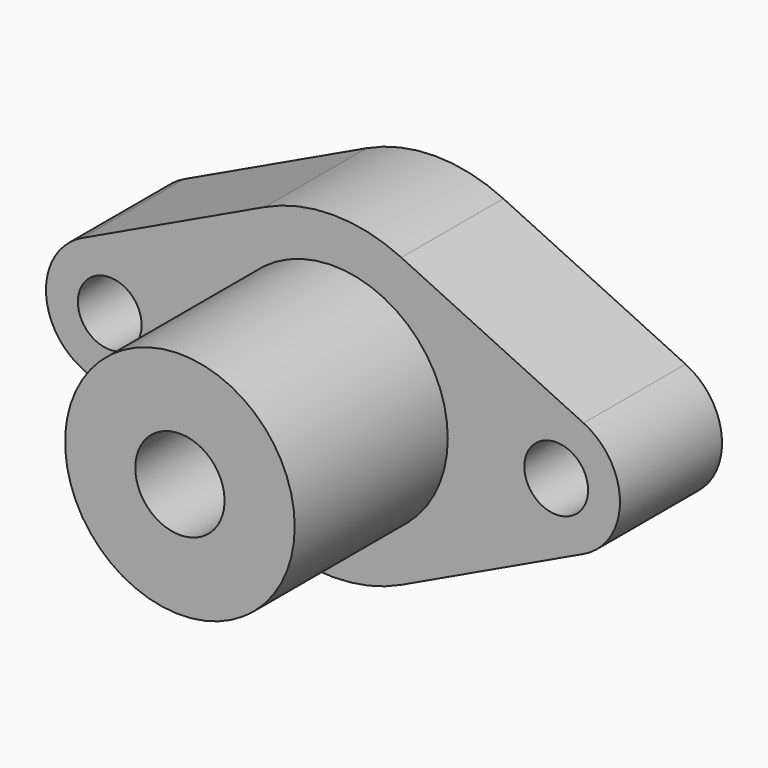
from build123d import *

# Parameters (mm, degrees)
F1_DEPTH    = 20
F2_T1_DEPTH = 125.4092553389
F3_D        = 10
F3_DEPTH    = 10
F3_TIP      = 3.0043030951
F4_R        = 18
F5_DEPTH    = 30
F7_D        = 14
F7_DEPTH    = 31
F7_TIP      = 4.2060243332
F8_T1_DEPTH = 79.2927061282


# Not quite as in the source:
# - a fillet or chamfer that OpenCascade refuses, or shapes differently, is made with other operations: its cross-section is extruded or revolved along the edge and cut away or added


with BuildPart() as f1:
    # F0 (on Front) → F1 (new body)
    with BuildSketch(Plane.XZ):
        with BuildLine():
            ThreePointArc((10.7142859294, -22.5876974706), (21.1288564318, -13.363061995), (25, 0))
            ThreePointArc((25, 0), (21.1288563814, 13.3630620747), (10.7142857589, 22.5876975515))
            ThreePointArc((10.7142857589, 22.5876975515), (1.61e-08, 25), (-10.7142857298, 22.5876975653))
            ThreePointArc((-10.7142857298, 22.5876975653), (-21.1288563728, 13.3630620884), (-25, 0))
            ThreePointArc((-25, 0), (-21.1288561313, -13.3630624702), (-10.7142849134, -22.5876979525))
            ThreePointArc((-10.7142849134, -22.5876979525), (5.623e-07, -25), (10.7142859294, -22.5876974706))
        make_face()
        with BuildLine():
            ThreePointArc((-39.2857140137, -9.0350791581), (-45, -4.32e-08), (-39.2857140918, 9.035079121))
            Line((-39.2857140918, 9.035079121), (-58.3333333333, 0))
            Line((-58.3333333333, 0), (-39.2857140137, -9.0350791581))
        make_face()
        with BuildLine():
            ThreePointArc((-25, 0), (-21.1288563728, 13.3630620884), (-10.7142857298, 22.5876975653))
            Line((-10.7142857298, 22.5876975653), (-39.2857140918, 9.035079121))
            ThreePointArc((-39.2857140918, 9.035079121), (-29.6547750711, 8.4515424899), (-25, 0))
        make_face()
        with BuildLine():
            Line((-39.2857140137, -9.0350791581), (-10.7142849134, -22.5876979525))
            ThreePointArc((-10.7142849134, -22.5876979525), (-21.1288561313, -13.3630624702), (-25, 0))
            ThreePointArc((-25, 0), (-29.6547750345, -8.4515424668), (-39.2857140137, -9.0350791581))
        make_face()
        with BuildLine():
            ThreePointArc((-39.2857140137, -9.0350791581), (-29.6547750345, -8.4515424668), (-25, 0))
            ThreePointArc((-25, 0), (-29.6547750711, 8.4515424899), (-39.2857140918, 9.035079121))
            ThreePointArc((-39.2857140918, 9.035079121), (-45, -4.32e-08), (-39.2857140137, -9.0350791581))
        make_face()
        with BuildLine():
            Line((0, -27.6699295265), (10.7142859294, -22.5876974706))
            ThreePointArc((10.7142859294, -22.5876974706), (5.623e-07, -25), (-10.7142849134, -22.5876979525))
            Line((-10.7142849134, -22.5876979525), (0, -27.6699295265))
        make_face()
        with BuildLine():
            ThreePointArc((-10.7142857298, 22.5876975653), (1.61e-08, 25), (10.7142857589, 22.5876975515))
            Line((10.7142857589, 22.5876975515), (0, 27.6699295265))
            Line((0, 27.6699295265), (-10.7142857298, 22.5876975653))
        make_face()
        with BuildLine():
            Line((58.3333333333, 0), (39.2857143013, 9.0350790217))
            ThreePointArc((39.2857143013, 9.0350790217), (43.4515425519, 5.345224831), (45, 0))
            ThreePointArc((45, 0), (43.4515424899, -5.3452249289), (39.2857140918, -9.035079121))
            Line((39.2857140918, -9.035079121), (58.3333333333, 0))
        make_face()
        with BuildLine():
            ThreePointArc((10.7142857589, 22.5876975515), (21.1288563814, 13.3630620747), (25, 0))
            ThreePointArc((25, 0), (29.654775169, 8.4515425519), (39.2857143013, 9.0350790217))
            Line((39.2857143013, 9.0350790217), (10.7142857589, 22.5876975515))
        make_face()
        with BuildLine():
            ThreePointArc((39.2857140918, -9.035079121), (29.6547750711, -8.4515424899), (25, 0))
            ThreePointArc((25, 0), (21.1288564318, -13.363061995), (10.7142859294, -22.5876974706))
            Line((10.7142859294, -22.5876974706), (39.2857140918, -9.035079121))
        make_face()
        with BuildLine():
            ThreePointArc((39.2857143013, 9.0350790217), (29.654775169, 8.4515425519), (25, 0))
            ThreePointArc((25, 0), (29.6547750711, -8.4515424899), (39.2857140918, -9.035079121))
            ThreePointArc((39.2857140918, -9.035079121), (43.4515424899, -5.3452249289), (45, 0))
            ThreePointArc((45, 0), (43.4515425519, 5.345224831), (39.2857143013, 9.0350790217))
        make_face()
    extrude(amount=-F1_DEPTH)

    # F2: fillet of radius 10 on 2 edges, made by hand

    # F2_s2 → F2_t1 (cut)
    with BuildSketch(Plane.XZ.offset(-72.7046276695)):
        with BuildLine():
            ThreePointArc((-39.2857142857, -9.0350790291), (-45, 0), (-39.2857142857, 9.0350790291))
            Line((-39.2857142857, 9.0350790291), (-58.3333333333, 0))
            Line((-58.3333333333, 0), (-39.2857142857, -9.0350790291))
        make_face()
        with BuildLine():
            ThreePointArc((39.2857142857, -9.0350790291), (45, 0), (39.2857142857, 9.0350790291))
            Line((39.2857142857, 9.0350790291), (58.3333333333, 0))
            Line((58.3333333333, 0), (39.2857142857, -9.0350790291))
        make_face()
    extrude(amount=F2_T1_DEPTH, mode=Mode.SUBTRACT)

    # F3
    with Locations(Plane.XZ):
        with Locations((-35, 0), (35, 0)):
            Hole(F3_D / 2, depth=F3_DEPTH)
            with Locations((0, 0, -(F3_DEPTH + F3_TIP / 2))):  # 118° drill point
                Cone(0, F3_D / 2, F3_TIP, mode=Mode.SUBTRACT)

    # F4 (on face) → F5 (join)
    with BuildSketch(Plane.XZ):
        Circle(F4_R)
    extrude(amount=F5_DEPTH)

    # F7
    with Locations(Plane.XZ.offset(30)):
        with Locations((0, 0)):
            Hole(F7_D / 2, depth=F7_DEPTH)
            with Locations((0, 0, -(F7_DEPTH + F7_TIP / 2))):  # 118° drill point
                Cone(0, F7_D / 2, F7_TIP, mode=Mode.SUBTRACT)

    # F8: fillet of radius 25 on 2 edges, made by hand

    # F8_s2 → F8_t1 (cut)
    with BuildSketch(Plane.XZ.offset(-49.6463530641)):
        with BuildLine():
            ThreePointArc((-10.7142857143, 22.5876975726), (0, 25), (10.7142857143, 22.5876975726))
            Line((10.7142857143, 22.5876975726), (0, 27.6699295265))
            Line((0, 27.6699295265), (-10.7142857143, 22.5876975726))
        make_face()
        with BuildLine():
            ThreePointArc((-10.7142857143, -22.5876975726), (0, -25), (10.7142857143, -22.5876975726))
            Line((10.7142857143, -22.5876975726), (0, -27.6699295265))
            Line((0, -27.6699295265), (-10.7142857143, -22.5876975726))
        make_face()
    extrude(amount=F8_T1_DEPTH, mode=Mode.SUBTRACT)


solid = f1.part
